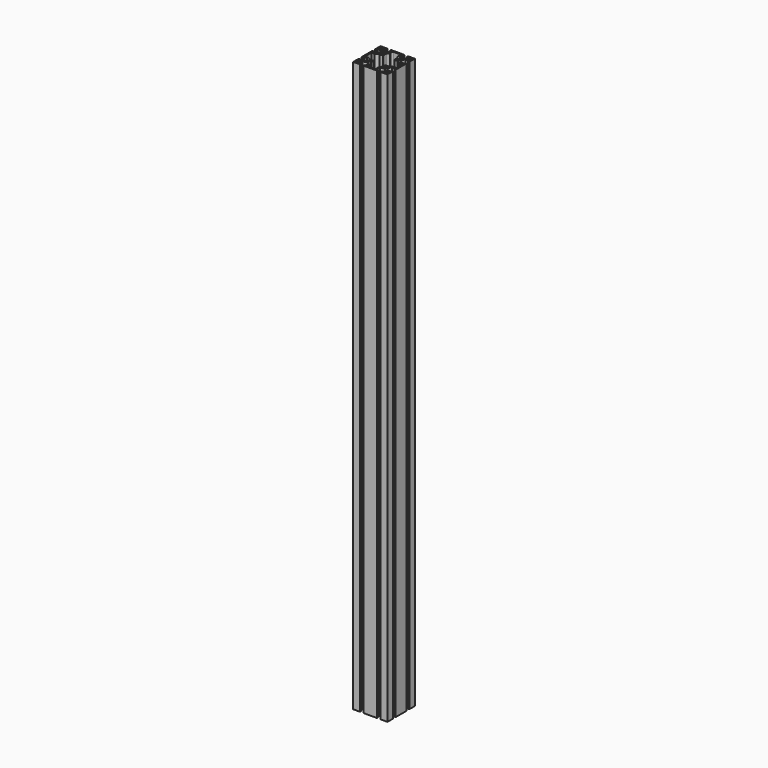
from build123d import *

# Parameters (mm, degrees)
F0_R     = 3
F0_R_2   = 2.5
F1_DEPTH = 1000
F2_R     = 2
F3_R     = 7


# Not quite as in the source:
# - a feature names something its author has since deleted; it is built from what else it names


with BuildPart() as f1:
    # F0 (on Top) → F1 (new body)
    with BuildSketch(Plane.XY):
        with BuildLine():
            Line((18.15, -30), (30, -30))
            Line((30, -30), (30, -18.15))
            Line((30, -18.15), (27.5, -18.15))
            Line((27.5, -18.15), (27.5, -20.15))
            Line((27.5, -20.15), (21.5477069044, -20.15))
            ThreePointArc((21.5477069044, -20.15), (19.5, -15), (21.5477069044, -9.85))
            Line((21.5477069044, -9.85), (27.5, -9.85))
            Line((27.5, -9.85), (27.5, -11.85))
            Line((27.5, -11.85), (30, -11.85))
            Line((30, -11.85), (30, 11.85))
            Line((30, 11.85), (27.5, 11.85))
            Line((27.5, 11.85), (27.5, 9.85))
            Line((27.5, 9.85), (21.5477069044, 9.85))
            ThreePointArc((21.5477069044, 9.85), (19.5, 15), (21.5477069044, 20.15))
            Line((21.5477069044, 20.15), (27.5, 20.15))
            Line((27.5, 20.15), (27.5, 18.15))
            Line((27.5, 18.15), (30, 18.15))
            Line((30, 18.15), (30, 30))
            Line((30, 30), (18.15, 30))
            Line((18.15, 30), (18.15, 27.5))
            Line((18.15, 27.5), (20.15, 27.5))
            Line((20.15, 27.5), (20.15, 21.5477069044))
            ThreePointArc((20.15, 21.5477069044), (15, 19.5), (9.85, 21.5477069044))
            Line((9.85, 21.5477069044), (9.85, 27.5))
            Line((9.85, 27.5), (11.85, 27.5))
            Line((11.85, 27.5), (11.85, 30))
            Line((11.85, 30), (-11.85, 30))
            Line((-11.85, 30), (-11.85, 27.5))
            Line((-11.85, 27.5), (-9.85, 27.5))
            Line((-9.85, 27.5), (-9.85, 21.5477069044))
            ThreePointArc((-9.85, 21.5477069044), (-15, 19.5), (-20.15, 21.5477069044))
            Line((-20.15, 21.5477069044), (-20.15, 27.5))
            Line((-20.15, 27.5), (-18.15, 27.5))
            Line((-18.15, 27.5), (-18.15, 30))
            Line((-18.15, 30), (-30, 30))
            Line((-30, 30), (-30, 18.15))
            Line((-30, 18.15), (-27.5, 18.15))
            Line((-27.5, 18.15), (-27.5, 20.15))
            Line((-27.5, 20.15), (-21.5477069044, 20.15))
            ThreePointArc((-21.5477069044, 20.15), (-19.5, 15), (-21.5477069044, 9.85))
            Line((-21.5477069044, 9.85), (-27.5, 9.85))
            Line((-27.5, 9.85), (-27.5, 11.85))
            Line((-27.5, 11.85), (-30, 11.85))
            Line((-30, 11.85), (-30, -11.85))
            Line((-30, -11.85), (-27.5, -11.85))
            Line((-27.5, -11.85), (-27.5, -9.85))
            Line((-27.5, -9.85), (-21.5477069044, -9.85))
            ThreePointArc((-21.5477069044, -9.85), (-19.5, -15), (-21.5477069044, -20.15))
            Line((-21.5477069044, -20.15), (-27.5, -20.15))
            Line((-27.5, -20.15), (-27.5, -18.15))
            Line((-27.5, -18.15), (-30, -18.15))
            Line((-30, -18.15), (-30, -30))
            Line((-30, -30), (-18.15, -30))
            Line((-18.15, -30), (-18.15, -27.5))
            Line((-18.15, -27.5), (-20.15, -27.5))
            Line((-20.15, -27.5), (-20.15, -21.5477069044))
            ThreePointArc((-20.15, -21.5477069044), (-15, -19.5), (-9.85, -21.5477069044))
            Line((-9.85, -21.5477069044), (-9.85, -27.5))
            Line((-9.85, -27.5), (-11.85, -27.5))
            Line((-11.85, -27.5), (-11.85, -30))
            Line((-11.85, -30), (11.85, -30))
            Line((11.85, -30), (11.85, -27.5))
            Line((11.85, -27.5), (9.85, -27.5))
            Line((9.85, -27.5), (9.85, -21.5477069044))
            ThreePointArc((9.85, -21.5477069044), (15, -19.5), (20.15, -21.5477069044))
            Line((20.15, -21.5477069044), (20.15, -27.5))
            Line((20.15, -27.5), (18.15, -27.5))
            Line((18.15, -27.5), (18.15, -30))
        make_face()
        with Locations((-25, -25)):
            Circle(F0_R, mode=Mode.SUBTRACT)
        with Locations((-15, -15)):
            Circle(F0_R_2, mode=Mode.SUBTRACT)
        with Locations((25, -25)):
            Circle(F0_R, mode=Mode.SUBTRACT)
        with Locations((15, -15)):
            Circle(F0_R_2, mode=Mode.SUBTRACT)
        with Locations((-25, 25)):
            Circle(F0_R, mode=Mode.SUBTRACT)
        with Locations((-15, 15)):
            Circle(F0_R_2, mode=Mode.SUBTRACT)
        Polygon((-7, 22), (-7, 27.5), (0, 27.5), (7, 27.5), (7, 22), (10, 16), (10, 10), (16, 10), (22, 7), (27.5, 7), (27.5, 0), (27.5, -7), (22, -7), (16, -10), (10, -10), (10, -16), (7, -22), (7, -27.5), (0, -27.5), (-7, -27.5), (-7, -22), (-10, -16), (-10, -10), (-16, -10), (-22, -7), (-27.5, -7), (-27.5, 0), (-27.5, 7), (-22, 7), (-16, 10), (-10, 10), (-10, 16), align=None, mode=Mode.SUBTRACT)
        with Locations((15, 15)):
            Circle(F0_R_2, mode=Mode.SUBTRACT)
        with Locations((25, 25)):
            Circle(F0_R, mode=Mode.SUBTRACT)
    extrude(amount=F1_DEPTH)

    # F2
    f2_edges = [f1.edges().sort_by_distance(p)[0] for p in [
        (-7, 27.5, 500),
        (7, 27.5, 500),
    ]]
    fillet(f2_edges, radius=F2_R)

    # F3
    f3_edges = [f1.edges().sort_by_distance(p)[0] for p in [
        (-10, 16, 500),
        (10, 16, 500),
    ]]
    fillet(f3_edges, radius=F3_R)


solid = f1.part
